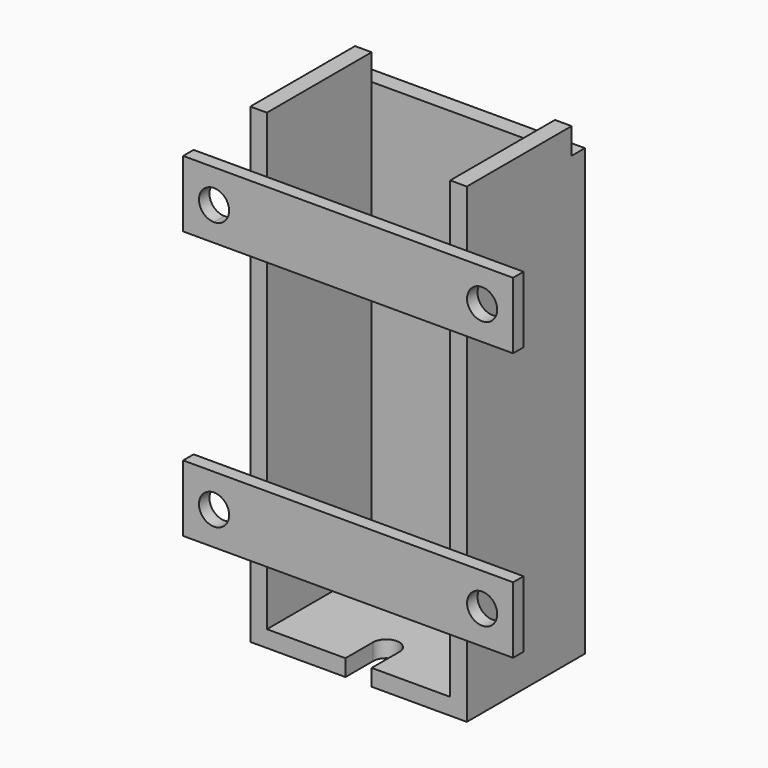
from build123d import *

# Parameters (mm, degrees)
F1_DEPTH  = 6.35
F2_W      = 50
F2_H      = 180
F3_DEPTH  = 6.35
F4_W      = 50
F4_H      = 180
F5_DEPTH  = 6.35
F6_W      = 70
F6_H      = 163.65
F7_DEPTH  = 6.35
F8_R      = 5.75
F8_W      = 6.35
F8_H      = 12.7
F8_W_2    = 30
F9_DEPTH  = 5
F11_DEPTH = 5


# Not quite as in the source:
# - a feature names something its author has since deleted; it is built from what else it names


with BuildPart() as f1:
    # F0 (on Top) → F1 (new body)
    with BuildSketch(Plane.XY):
        with BuildLine():
            Line((35, -25), (35, 25))
            Line((35, 25), (-35, 25))
            Line((-35, 25), (-35, -25))
            Line((-35, -25), (-5, -25))
            Line((-5, -25), (-5, -11.8))
            ThreePointArc((-5, -11.8), (0, -6.8), (5, -11.8))
            Line((5, -11.8), (5, -25))
            Line((5, -25), (35, -25))
        make_face()
    extrude(amount=F1_DEPTH)

    # F2 (on face) → F3 (join)
    with BuildSketch(Plane(origin=(-35, 0, 0), x_dir=(0, -1, 0), z_dir=(-1, 0, 0))):
        with Locations((0, 90)):
            Rectangle(F2_W, F2_H)
    extrude(amount=F3_DEPTH)

    # F4 (on face) → F5 (join)
    with BuildSketch(Plane.YZ.offset(35)):
        with Locations((0, 90)):
            Rectangle(F4_W, F4_H)
    extrude(amount=F5_DEPTH)

    # F6 (on face) → F7 (join)
    with BuildSketch(Plane(origin=(0, 25, 0), x_dir=(-1, 0, 0), z_dir=(0, 1, 0))):
        with Locations((0, 88.175)):
            Rectangle(F6_W, F6_H)
        Polygon((-41.35, 0), (41.35, 0), (41.35, 170), (35, 170), (35, 6.35), (-35, 6.35), (-35, 170), (-41.35, 170), align=None)
    extrude(amount=F7_DEPTH)

    # F8 (on face) → F9 (join)
    with BuildSketch(Plane.XZ.offset(25)):
        Polygon((-63, 30.625), (-5, 30.625), (-5, 43.325), (-5, 56.025), (-63, 56.025), align=None)
        with Locations((-51.19, 43.325)):
            Circle(F8_R, mode=Mode.SUBTRACT)
        Polygon((-5, 30.625), (5, 30.625), (5, 43.325), (5, 56.025), (-5, 56.025), (-5, 43.325), align=None)
        Polygon((41.35, 43.325), (41.35, 30.625), (63, 30.625), (63, 56.025), (41.35, 56.025), align=None)
        with BuildLine():
            ThreePointArc((56.94, 43.325), (51.19, 37.575), (45.44, 43.325))
            ThreePointArc((45.44, 43.325), (51.19, 49.075), (56.94, 43.325))
        make_face(mode=Mode.SUBTRACT)
        with Locations((38.175, 49.675)):
            Rectangle(F8_W, F8_H)
        with Locations((38.175, 36.975)):
            Rectangle(F8_W, F8_H)
        with Locations((20, 36.975)):
            Rectangle(F8_W_2, F8_H)
        with Locations((20, 49.675)):
            Rectangle(F8_W_2, F8_H)
    extrude(amount=F9_DEPTH)

    # F10 (on face) → F11 (join)
    with BuildSketch(Plane.XZ.offset(30)):
        Polygon((-63, 132.995), (-51.19, 132.995), (63, 132.995), (63, 158.395), (-63, 158.395), align=None)
        with BuildLine():
            ThreePointArc((-45.44, 145.695), (-47.1241360082, 141.6291360082), (-51.19, 139.945))
            ThreePointArc((-51.19, 139.945), (-55.2558639918, 149.7608639918), (-45.44, 145.695))
        make_face(mode=Mode.SUBTRACT)
        with BuildLine():
            ThreePointArc((56.93, 145.695), (51.18, 139.945), (45.43, 145.695))
            ThreePointArc((45.43, 145.695), (51.18, 151.445), (56.93, 145.695))
        make_face(mode=Mode.SUBTRACT)
    extrude(amount=-F11_DEPTH)


solid = f1.part
